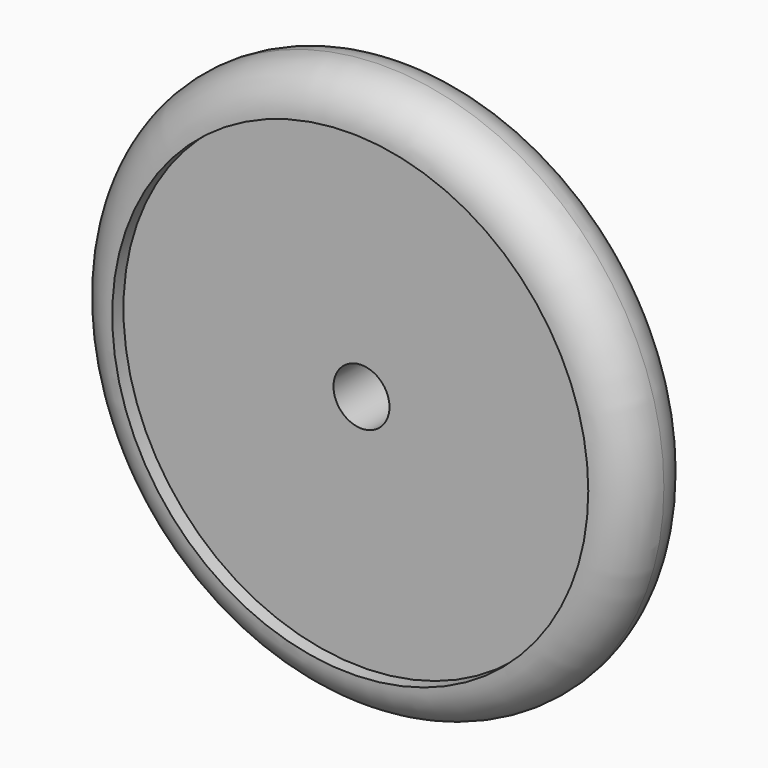
from build123d import *

# Parameters (mm, degrees)
F0_R     = 100
F1_DEPTH = 30
F2_R     = 14.99999
F3_DEPTH = 5
F4_R     = 10
F5_DEPTH = 25.001


# Not quite as in the source:
# - a fillet or chamfer is up to 0.001 mm smaller than in the source, because OpenCascade refuses the exact size


with BuildPart() as f1:
    # F0 (on Front) → F1 (new body)
    with BuildSketch(Plane.XZ):
        Circle(F0_R)
    extrude(amount=F1_DEPTH)

    # F2 (radius 15 in the source; OpenCascade refuses exactly that, so slightly less here)
    f2_edges = [f1.edges().sort_by_distance(p)[0] for p in [
        (-100, -30, 0),
        (-100, 0, 0),
    ]]
    fillet(f2_edges, radius=F2_R)

    # F3 (cut): a face of the model
    f3_faces = [f1.faces().sort_by_distance(p)[0] for p in [
        (0, -30, 0),
    ]]
    extrude(f3_faces, amount=-F3_DEPTH, mode=Mode.SUBTRACT)

    # F4 (on face) → F5 (cut, through all)
    with BuildSketch(Plane.XZ.offset(25)):
        Circle(F4_R)
    extrude(amount=-F5_DEPTH, mode=Mode.SUBTRACT)


solid = f1.part
